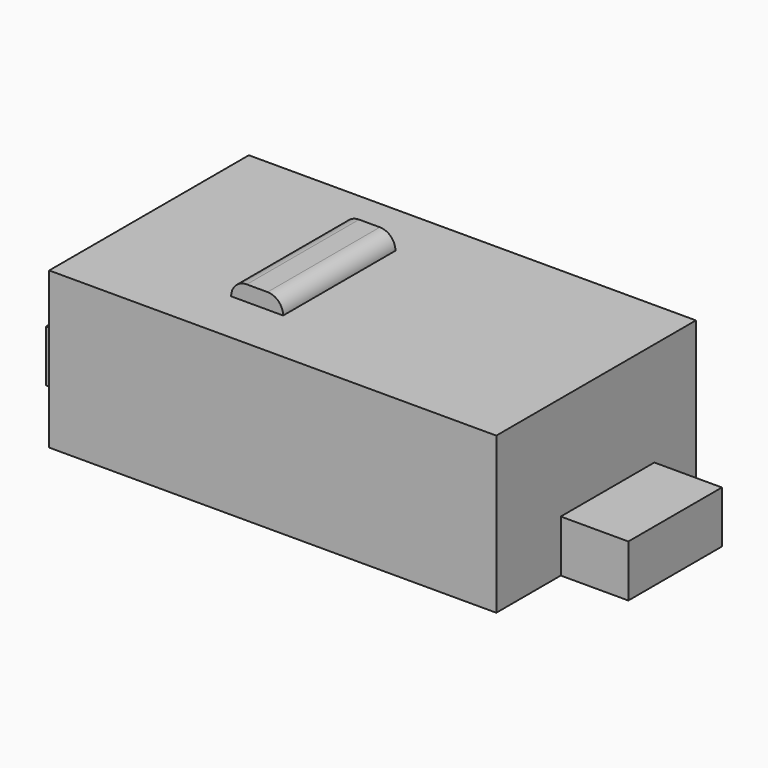
from build123d import *

# Parameters (mm, degrees)
F0_W     = 8.6
F0_H     = 4.8
F1_DEPTH = 3
F2_R     = 0.475
F3_DEPTH = 0.6
F4_SIZE  = 0.2
F5_W     = 1.3
F5_H     = 2.25
F6_DEPTH = 1
F7_W     = 1
F7_H     = 2.7
F8_DEPTH = 0.3
F9_R     = 0.29999


# Not quite as in the source:
# - a fillet or chamfer is up to 0.001 mm smaller than in the source, because OpenCascade refuses the exact size


with BuildPart() as f1:
    # F0 (on Top) → F1 (new body)
    with BuildSketch(Plane.XY):
        Rectangle(F0_W, F0_H)
    extrude(amount=F1_DEPTH)

    # F2 (on face) → F3 (join)
    with BuildSketch(Plane(origin=(0, 0, 0), x_dir=(1, 0, 0), z_dir=(0, 0, -1))):
        with Locations((-2, 0)):
            Circle(F2_R)
        with Locations((2, 0)):
            Circle(F2_R)
    extrude(amount=F3_DEPTH)

    # F4
    f4_edges = [f1.edges().sort_by_distance(p)[0] for p in [
        (-2.475, 0, -0.6),
        (1.525, 0, -0.6),
    ]]
    chamfer(f4_edges, length=F4_SIZE)

    # F5 (on Top) → F6 (join)
    with BuildSketch(Plane.XY):
        with Locations((-4.95, 0.275)):
            Rectangle(F5_W, F5_H)
        with Locations((4.95, 0.275)):
            Rectangle(F5_W, F5_H)
    extrude(amount=F6_DEPTH)

    # F7 (on face) → F8 (join)
    with BuildSketch(Plane.XY.offset(3)):
        with Locations((-1.14, 0)):
            Rectangle(F7_W, F7_H)
    extrude(amount=F8_DEPTH)

    # F9 (radius 0.3 in the source; OpenCascade refuses exactly that, so slightly less here)
    f9_edges = [f1.edges().sort_by_distance(p)[0] for p in [
        (-1.64, 0, 3.3),
        (-0.64, 0, 3.3),
    ]]
    fillet(f9_edges, radius=F9_R)


with BuildPart() as f1_1:
    # F10: moved
    add(f1.part.moved(Location((1.14, 0, 0))))


solid = f1_1.part
